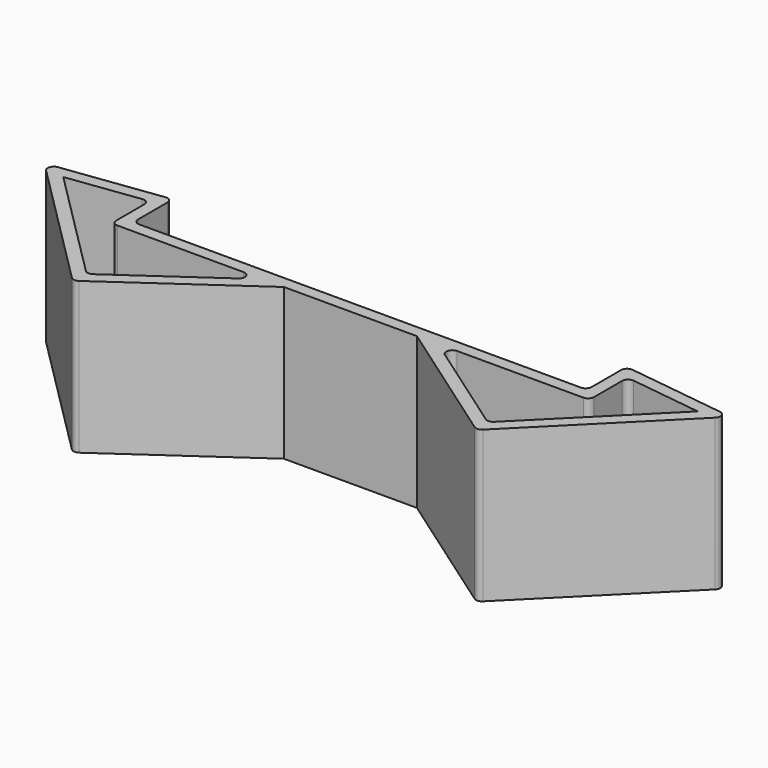
from build123d import *

# Parameters (mm, degrees)
F1_DEPTH = 25
F2_R     = 1


# Not quite as in the source:
# - a feature names something its author has since deleted; it is built from what else it names


with BuildPart() as f1:
    # F0 (on Top) → F1 (new body)
    with BuildSketch(Plane.XY):
        Polygon((0, -2), (0, 0), (-37.5, 0), (-37.5, 8.1967763358), (-56.72952592, 5.6744525365), (-33.382604787, -17.6724685966), (-11, -2), align=None)
        Polygon((-39.5, -2), (-14.4868935912, -2), (-33.1550573032, -15.0715889556), (-52.4458532095, 4.2192069507), (-39.5, 5.9173056865), align=None, mode=Mode.SUBTRACT)
        Polygon((37.5, 0), (0, 0), (0, -2), (11, -2), (33.382604787, -17.6724685966), (56.72952592, 5.6744525365), (37.5, 8.1967763358), align=None)
        Polygon((33.1550573032, -15.0715889556), (14.4868935912, -2), (39.5, -2), (39.5, 5.9173056865), (52.4458532095, 4.2192069507), align=None, mode=Mode.SUBTRACT)
    extrude(amount=F1_DEPTH)

    # F2
    f2_edges = [f1.edges().sort_by_distance(p)[0] for p in [
        (-37.5, 8.196776, 12.5),
        (-56.729526, 5.674453, 12.5),
        (-33.382605, -17.672469, 12.5),
        (-37.5, 0, 12.5),
        (-39.5, -2, 12.5),
        (37.5, 0, 12.5),
        (37.5, 8.196776, 12.5),
        (56.729526, 5.674453, 12.5),
        (39.5, -2, 12.5),
        (33.382605, -17.672469, 12.5),
        (14.486894, -2, 12.5),
        (-14.486894, -2, 12.5),
        (-39.5, 5.917306, 12.5),
        (-33.155057, -15.071589, 12.5),
        (39.5, 5.917306, 12.5),
        (33.155057, -15.071589, 12.5),
    ]]
    fillet(f2_edges, radius=F2_R)


solid = f1.part
